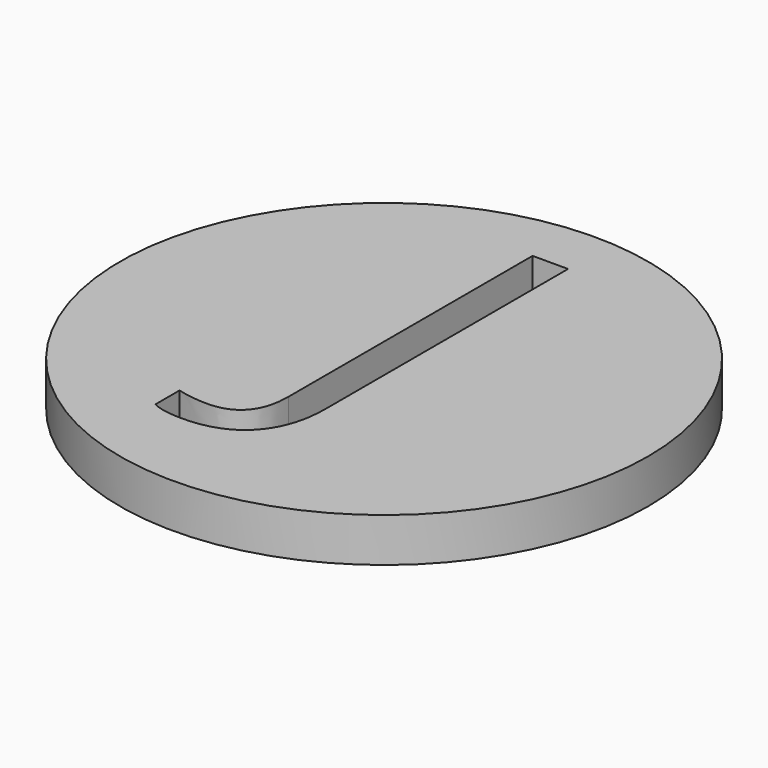
from build123d import *

# Parameters (mm, degrees)
F0_R         = 12
F1_DEPTH     = 2
F2_TEXT_SIZE = 19.4444444444
F3_DEPTH     = 25


# Not quite as in the source:
# - Text() gives the source's letters only with a copy of the font that has no kerning and outlines rounded to 1/6400 em; it was checked with that copy


with BuildPart() as f1:
    # F0 (on Top) → F1 (new body)
    with BuildSketch(Plane.XY):
        Circle(F0_R)
    extrude(amount=F1_DEPTH)

    # F2 (on face) → F3 (cut)
    with BuildSketch(Plane.XY.offset(2)):
        with Locations((-2.6414076565, -4.3979441151)):
            Text('J', F2_TEXT_SIZE, font='Open Sans', text_align=(TextAlign.LEFT, TextAlign.BOTTOM))
    extrude(amount=-F3_DEPTH, mode=Mode.SUBTRACT)


solid = f1.part
